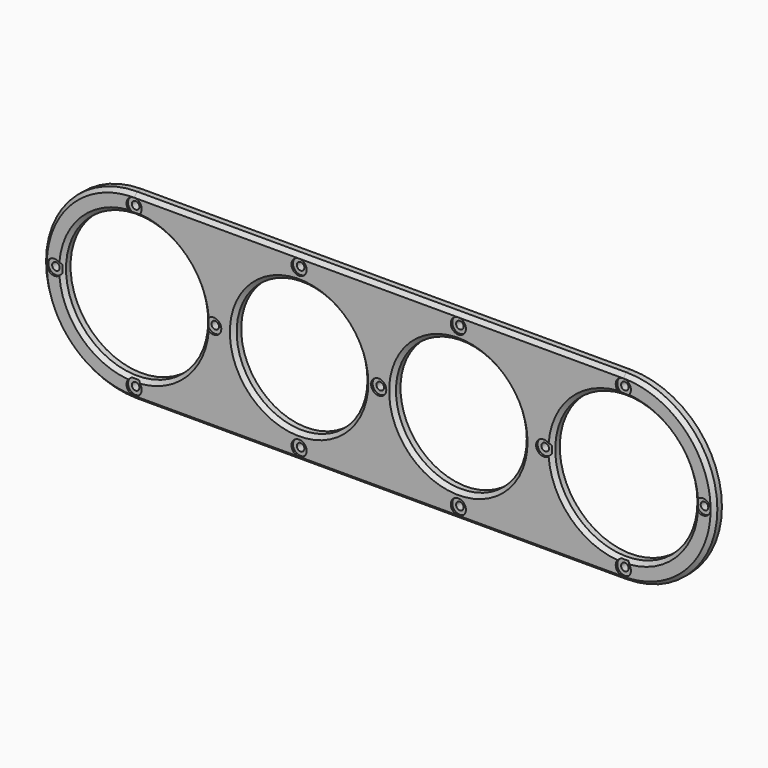
from build123d import *

# Parameters (mm, degrees)
F0_R     = 2
F0_R_2   = 37.5
F0_R_3   = 34.5
F1_DEPTH = 5
F2_SIZE  = 2
F3_SIZE  = 2
F4_R     = 4
F5_DEPTH = 1
F6_SIZE  = 1.99999


# Not quite as in the source:
# - a fillet or chamfer is up to 0.001 mm smaller than in the source, because OpenCascade refuses the exact size


with BuildPart() as f1:
    # F0 (on Front) → F1 (new body)
    with BuildSketch(Plane.XZ):
        with BuildLine():
            ThreePointArc((129, -48), (177, 0), (129, 48))
            Line((129, 48), (0, 48))
            Line((0, 48), (-129, 48))
            ThreePointArc((-129, 48), (-177, 0), (-129, -48))
            Line((-129, -48), (0, -48))
            Line((0, -48), (129, -48))
        make_face()
        with Locations((-129, -42)):
            Circle(F0_R, mode=Mode.SUBTRACT)
        with Locations((-42, -42)):
            Circle(F0_R, mode=Mode.SUBTRACT)
        with Locations((42, -42)):
            Circle(F0_R, mode=Mode.SUBTRACT)
        with Locations((129, -42)):
            Circle(F0_R, mode=Mode.SUBTRACT)
        with Locations((-171, 0)):
            Circle(F0_R, mode=Mode.SUBTRACT)
        with Locations((-129, 0)):
            Circle(F0_R_2, mode=Mode.SUBTRACT)
        with Locations((-87, 0)):
            Circle(F0_R, mode=Mode.SUBTRACT)
        with Locations((-42, 0)):
            Circle(F0_R_3, mode=Mode.SUBTRACT)
        with Locations((-129, 42)):
            Circle(F0_R, mode=Mode.SUBTRACT)
        with Locations((-42, 42)):
            Circle(F0_R, mode=Mode.SUBTRACT)
        Circle(F0_R, mode=Mode.SUBTRACT)
        with Locations((42, 0)):
            Circle(F0_R_3, mode=Mode.SUBTRACT)
        with Locations((87, 0)):
            Circle(F0_R, mode=Mode.SUBTRACT)
        with Locations((129, 0)):
            Circle(F0_R_2, mode=Mode.SUBTRACT)
        with Locations((171, 0)):
            Circle(F0_R, mode=Mode.SUBTRACT)
        with Locations((42, 42)):
            Circle(F0_R, mode=Mode.SUBTRACT)
        with Locations((129, 42)):
            Circle(F0_R, mode=Mode.SUBTRACT)
    extrude(amount=F1_DEPTH)

    # F2
    f2_edges = [f1.edges().sort_by_distance(p)[0] for p in [
        (7.5, -5, 0),
        (-76.5, -5, 0),
    ]]
    chamfer(f2_edges, length=F2_SIZE)

    # F3
    f3_edges = [f1.edges().sort_by_distance(p)[0] for p in [
        (91.5, -5, 0),
        (-166.5, -5, 0),
    ]]
    chamfer(f3_edges, length=F3_SIZE)

    # F4 (on face) → F5 (cut)
    with BuildSketch(Plane.XZ.offset(5)):
        Circle(F4_R)
        with Locations((42, 42)):
            Circle(F4_R)
        with Locations((42, -42)):
            Circle(F4_R)
        with Locations((129, 42)):
            Circle(F4_R)
        with Locations((87, 0)):
            Circle(F4_R)
        with Locations((129, -42)):
            Circle(F4_R)
        with Locations((171, 0)):
            Circle(F4_R)
        with Locations((-42, 42)):
            Circle(F4_R)
        with Locations((-42, -42)):
            Circle(F4_R)
        with Locations((-87, 0)):
            Circle(F4_R)
        with Locations((-129, -42)):
            Circle(F4_R)
        with Locations((-129, 42)):
            Circle(F4_R)
        with Locations((-171, 0)):
            Circle(F4_R)
    extrude(amount=-F5_DEPTH, mode=Mode.SUBTRACT)

    # F6 (size 2 in the source; OpenCascade refuses exactly that, so slightly less here)
    f6_edges = [f1.edges().sort_by_distance(p)[0] for p in [
        (-177, -5, 0),
        (0, -5, 48),
        (0, -5, -48),
        (177, -5, 0),
    ]]
    chamfer(f6_edges, length=F6_SIZE)


solid = f1.part
